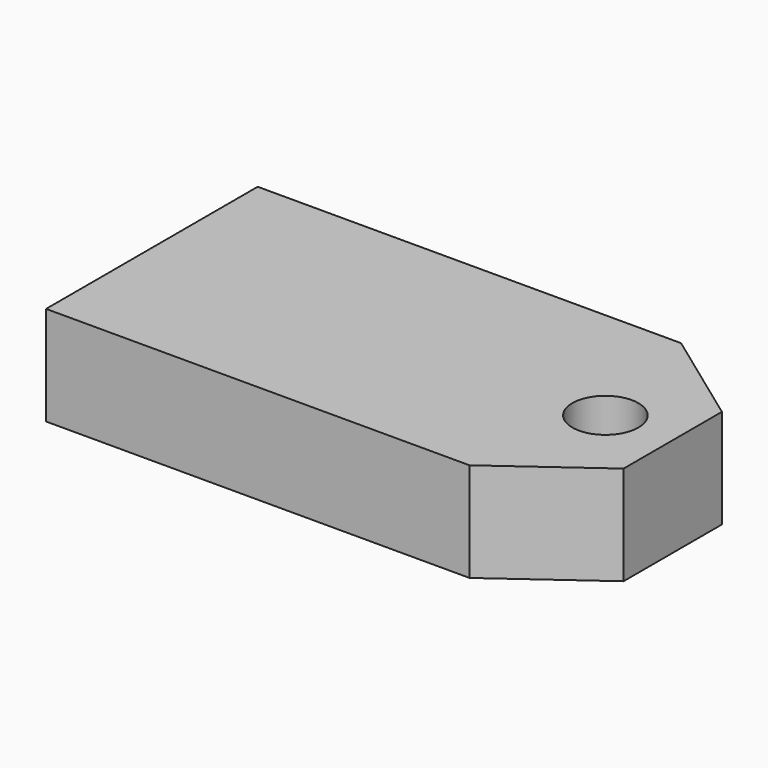
from build123d import *

# Parameters (mm, degrees)
F0_R         = 3.175
F1_DEPTH     = 9.525
F2_TEXT_SIZE = 9.0798733942
F3_DEPTH     = 3.175


# Not quite as in the source:
# - Text() gives the source's letters only with a copy of the font that has no kerning and outlines rounded to 1/6400 em; it was checked with that copy


with BuildPart() as f1:
    # F0 (on Top) → F1 (new body)
    with BuildSketch(Plane.XY):
        Polygon((-15.2667295207, -13.0267653942), (-15.2667295207, -25.7267653942), (-15.2667295207, -38.4267653942), (25.395551737, -38.4267653942), (34.7534483983, -31.6311512094), (34.7534483983, -25.7267653942), (34.7534483983, -19.822379579), (25.395551737, -13.0267653942), align=None)
        with Locations((28.286146, -25.7267653942)):
            Circle(F0_R, mode=Mode.SUBTRACT)
    extrude(amount=F1_DEPTH)

    # F2 (on face) → F3 (cut)
    with BuildSketch(Plane.XY.offset(9.525)):
        with Locations((-56.6051469694, -37.4110749785)):
            Text('Punahou', F2_TEXT_SIZE, font='Open Sans', text_align=(TextAlign.LEFT, TextAlign.BOTTOM))
    extrude(amount=-F3_DEPTH, mode=Mode.SUBTRACT)


solid = f1.part
